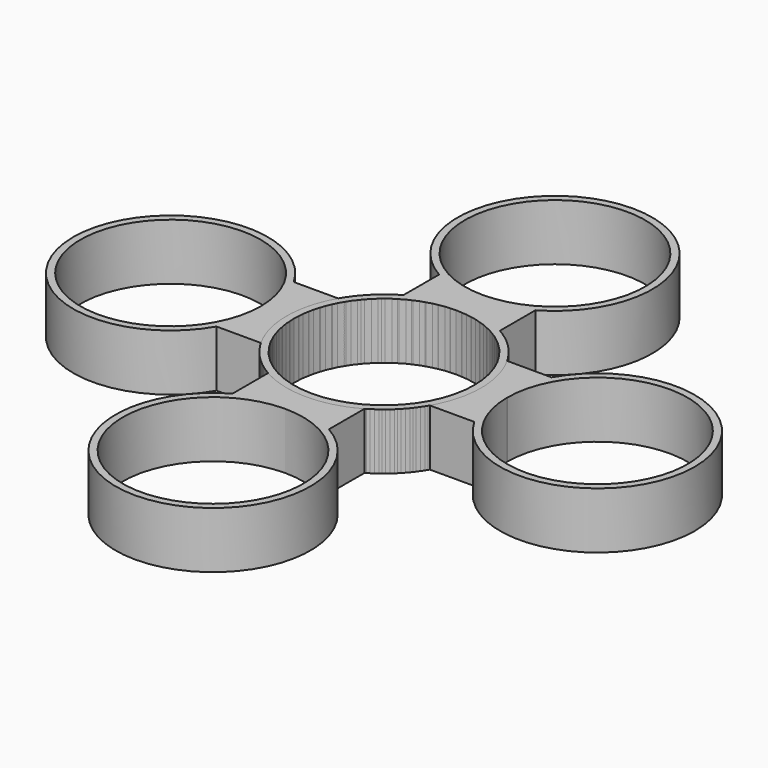
from build123d import *

# Parameters (mm, degrees)
F1_DEPTH        = 7
F1_COPIES_COUNT = 4


# Not quite as in the source:
# - a pattern or mirror of a feature is missing from the dataset's text; its kind, count and spacing are read off the source's solid
# - a feature names something its author has since deleted; it is built from what else it names


with BuildPart() as f1:
    # F0 (on Top) → F1 (new body)
    with BuildSketch(Plane.XY):
        with BuildLine():
            ThreePointArc((-10.4742522057, 5.9878431619), (-11.6594433384, 3.1018713769), (-12.0649970161, 0.0084853068))
            ThreePointArc((-12.0649970161, 0.0084853068), (-11.6637948914, -3.0854681543), (-10.4826643344, -5.9731041722))
            ThreePointArc((-10.4826643344, -5.9731041722), (3.0895695335, -11.6627091663), (12.065, 0))
            ThreePointArc((12.065, 0), (3.0977711454, 11.6605333896), (-10.4742522057, 5.9878431619))
        make_face()
        with BuildLine():
            ThreePointArc((-11.1749972363, 0.0078593704), (0.0039296854, 11.1749993091), (11.175, 0))
            ThreePointArc((11.175, 0), (-0.0039296854, -11.1749993091), (-11.1749972363, 0.0078593704))
        make_face(mode=Mode.SUBTRACT)
        with BuildLine():
            ThreePointArc((-10.4826643344, -5.9731041722), (-11.6637948914, -3.0854681543), (-12.0649970161, 0.0084853068))
            Line((-12.0649970161, 0.0084853068), (-14.3983957949, 0.0101263851))
            ThreePointArc((-14.3983957949, 0.0101263851), (-14.8033767561, -3.0811061337), (-15.9869294116, -5.9653618742))
            Line((-15.9869294116, -5.9653618742), (-10.4826643344, -5.9731041722))
        make_face()
        with BuildLine():
            Line((-14.3983957949, 0.0101263851), (-12.0649970161, 0.0084853068))
            ThreePointArc((-12.0649970161, 0.0084853068), (-11.6594433384, 3.1018713769), (-10.4742522057, 5.9878431619))
            Line((-10.4742522057, 5.9878431619), (-15.978522728, 5.9878431619))
            ThreePointArc((-15.978522728, 5.9878431619), (-14.8001132004, 3.1060270712), (-14.398392811, 0.0186116919))
            ThreePointArc((-14.398392811, 0.0186116919), (-14.398393557, 0.0143690382), (-14.3983957949, 0.0101263851))
        make_face()
        with BuildLine():
            ThreePointArc((-15.9869294116, -5.9653618742), (-14.8033767561, -3.0811061337), (-14.3983957949, 0.0101263851))
            ThreePointArc((-14.3983957949, 0.0101263851), (-14.398393557, 0.0143690382), (-14.398392811, 0.0186116919))
            ThreePointArc((-14.398392811, 0.0186116919), (-14.8001132004, 3.1060270712), (-15.978522728, 5.9878431619))
            ThreePointArc((-15.978522728, 5.9878431619), (-38.5283898272, 0.0270969987), (-15.9869294116, -5.9653618742))
        make_face()
        with BuildLine():
            ThreePointArc((-15.288392811, 0.0186116919), (-15.288393502, 0.0146820065), (-15.2883955748, 0.0107523215))
            ThreePointArc((-15.2883955748, 0.0107523215), (-37.6383921201, 0.0225413774), (-15.288392811, 0.0186116919))
        make_face(mode=Mode.SUBTRACT)
    extrude(amount=F1_DEPTH)


with BuildPart() as f1_copies_1:
    # F1_copies: instance of F1
    add(f1.part.rotate(Axis((0, 0, 0), (0, 0, 1)), 1 * 360 / F1_COPIES_COUNT))


with BuildPart() as f1_copies_2:
    # F1_copies: instance of F1
    add(f1.part.rotate(Axis((0, 0, 0), (0, 0, 1)), 2 * 360 / F1_COPIES_COUNT))


with BuildPart() as f1_copies_3:
    # F1_copies: instance of F1
    add(f1.part.rotate(Axis((0, 0, 0), (0, 0, 1)), 3 * 360 / F1_COPIES_COUNT))


solid = Compound([f1.part, f1_copies_1.part, f1_copies_2.part, f1_copies_3.part])
